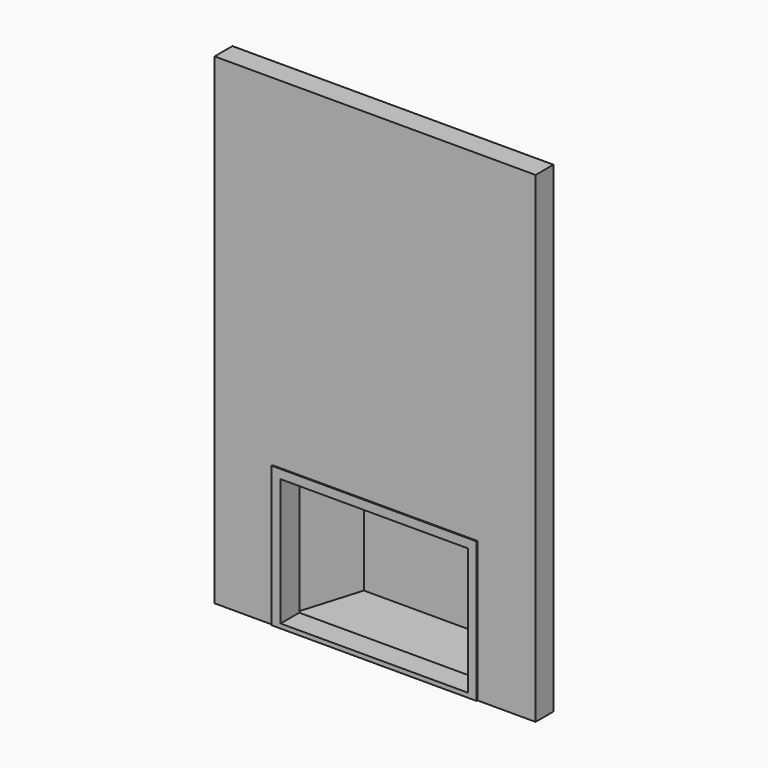
from build123d import *

# Parameters (mm, degrees)
F0_W          = 1828.8
F0_H          = 2743.2
F1_DEPTH      = 127
F2_W          = 1168.4
F2_H          = 800.1
F2_W_2        = 1066.8
F2_H_2        = 723.9
F3_DEPTH      = 508
F3_DEPTH_BACK = 6.35
F5_DEPTH      = 800.101
F6_W          = 1066.8
F6_H          = 723.9
F7_DEPTH      = 133.35
F8_T          = -6.35


# Not quite as in the source:
# - a shell that OpenCascade refuses in one call is made with other operations: the cavity is built on its own and cut out


with BuildPart() as f1:
    # F0 (on Front) → F1 (new body)
    with BuildSketch(Plane.XZ):
        Rectangle(F0_W, F0_H)
    extrude(amount=F1_DEPTH)

    # F2 (on face) → F3 (join, two sides)
    with BuildSketch(Plane.XZ.offset(127)) as f3_sk:
        with Locations((0, -971.55)):
            Rectangle(F2_W, F2_H)
        with Locations((0, -984.25)):
            Rectangle(F2_W_2, F2_H_2, mode=Mode.SUBTRACT)
        with Locations((0, -984.25)):
            Rectangle(F2_W_2, F2_H_2)
    extrude(amount=-F3_DEPTH)
    extrude(f3_sk.sketch, amount=F3_DEPTH_BACK)

    # F4 (on face) → F5 (cut, through all)
    with BuildSketch(Plane.XY.offset(-571.5)):
        Polygon((-469.9, 381), (-584.2, 381), (-584.2, 0), align=None)
        Polygon((584.2, 381), (469.9, 381), (584.2, 0), align=None)
    extrude(amount=-F5_DEPTH, mode=Mode.SUBTRACT)

    # F6 (on face) → F7 (cut)
    with BuildSketch(Plane.XZ.offset(133.35)):
        with Locations((0, -984.25)):
            Rectangle(F6_W, F6_H)
    extrude(amount=-F7_DEPTH, mode=Mode.SUBTRACT)

    # F8: a shell. OpenCascade refuses it in one call, so the cavity is built on its own and cut out:
    # the body offset inwards by the wall thickness, plus a prism from it out through each open face.
    f8_core = offset(f1.part, amount=F8_T, kind=Kind.INTERSECTION, mode=Mode.PRIVATE)
    f8_exits = [f8_core.faces().sort_by_distance(p)[0] for p in [
        (0, 6.35, -984.25),
    ]]
    add(f8_core, mode=Mode.SUBTRACT)
    extrude(f8_exits, amount=-F8_T, mode=Mode.SUBTRACT)


solid = f1.part
